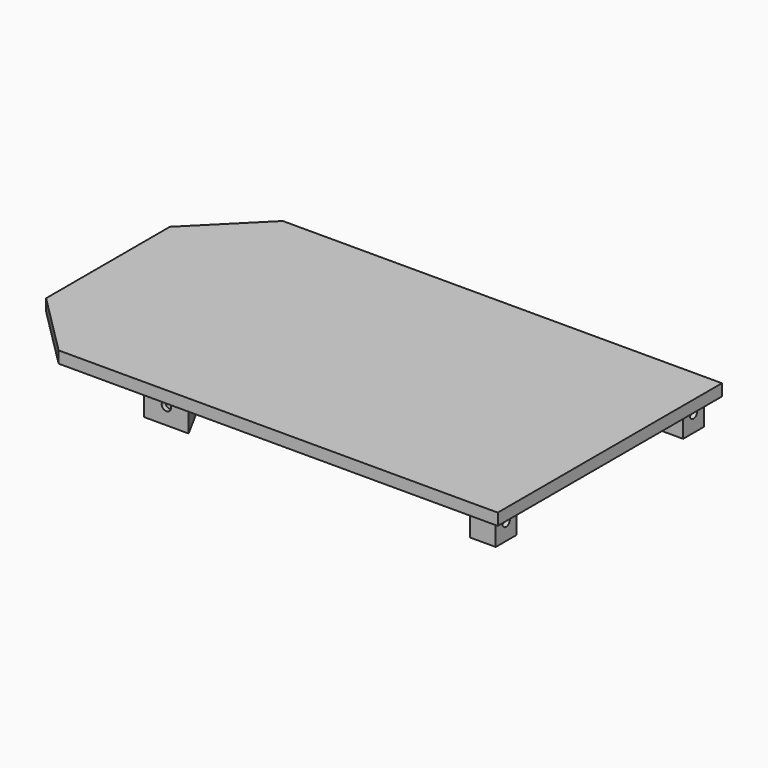
from build123d import *

# Parameters (mm, degrees)
F0_W      = 7.8739928325
F0_H      = 7.8739928325
F1_DEPTH  = 2.54
F2_DEPTH  = 1.016
F3_DEPTH  = 8.89
F8_W      = 2.286
F8_H      = 6.35
F7_W      = 2.286
F7_H      = 6.35
F4_W      = 6.35
F4_H      = 2.286
F5_W      = 2.286
F5_H      = 6.35
F6_W      = 6.35
F6_H      = 2.286
F9_DEPTH  = 8.255
F10_R     = 1.4224
F11_DEPTH = 101.6
F12_R     = 1.4224
F13_R     = 1.4224
F14_DEPTH = 25.4
F15_R     = 1.4224
F16_DEPTH = 25.4


# Not quite as in the source:
# - a feature names something its author has since deleted; it is built from what else it names


with BuildPart() as f1:
    # F0 (on Top) → F1 (new body)
    with BuildSketch(Plane.XY):
        Polygon((-50.5911594971, 45.1345390935), (-65.0638575705, 30.6618410202), (-69.6408525109, 26.0848460797), (-69.6408525109, 9.5127671957), (-69.6408525109, -20.9057678927), (-62.6880467633, -27.8585736403), (-50.5911594971, -39.9554609065), (82.7588405029, -39.9554609065), (82.7588405029, -17.0967224985), (82.7588405029, 43.8645390935), (82.7588405029, 45.1345390935), (33.1444106996, 45.1345390935), (-20.2568043023, 45.1345390935), align=None)
        Polygon((-50.0651082729, -38.6854609065), (-68.3711594971, -20.3794096823), (-68.3711594971, 25.5584878693), (-64.1658319583, 29.763815408), (-50.0651082729, 43.8645390935), (81.4888405029, 43.8645390935), (81.4888405029, -38.6854609065), align=None, mode=Mode.SUBTRACT)
        Polygon((-68.3711594971, 25.5584878693), (-68.3711594971, -20.3794096823), (-50.0651082729, -38.6854609065), (81.4888405029, -38.6854609065), (81.4888405029, 43.8645390935), (-50.0651082729, 43.8645390935), (-64.1658319583, 29.763815408), align=None)
        Polygon((-13.562855112, -36.9074608927), (-27.0518330949, -36.9074608927), (-22.3274411258, -29.0334609202), (-17.8373202542, -29.0334609202), align=None, mode=Mode.SUBTRACT)
        Polygon((-66.5931594971, -19.6429379684), (-66.5931594971, -12.7413552397), (-60.0190392027, -12.7413552397), (-60.413067775, -19.6310556945), (-63.509054773, -22.7270426925), align=None, mode=Mode.SUBTRACT)
        with BuildLine():
            Line((-49.5390570487, -37.4154609065), (-61.7130058245, -25.2415121307))
            Line((-61.7130058245, -25.2415121307), (-58.120903376, -21.6494096823))
            Line((-58.120903376, -21.6494096823), (-56.9411594971, -12.2333584581))
            Line((-56.9411594971, -12.2333584581), (-56.9411594971, -9.6933584581))
            Line((-56.9411594971, -9.6933584581), (-67.1011594971, -9.6933584581))
            Line((-67.1011594971, -9.6933584581), (-67.1011594971, 25.0324366451))
            Line((-67.1011594971, 25.0324366451), (-49.5390570487, 42.5945390935))
            Line((-49.5390570487, 42.5945390935), (-33.3653066841, 42.5945390935))
            ThreePointArc((-33.3653066841, 42.5945390935), (-30.8623950498, 41.9351536832), (-29.0092406655, 40.128174271))
            Line((-29.0092406655, 40.128174271), (-25.1550660971, 33.7045390935))
            ThreePointArc((-25.1550660971, 33.7045390935), (-23.284234992, 31.8649136199), (-20.7556570459, 31.1645390935))
            Line((-20.7556570459, 31.1645390935), (-19.3944751483, 31.1645390935))
            ThreePointArc((-19.3944751483, 31.1645390935), (-16.8544751483, 31.8451300423), (-14.9950660971, 33.7045390935))
            Line((-14.9950660971, 33.7045390935), (-11.6110890868, 39.9381692669))
            ThreePointArc((-11.6110890868, 39.9381692669), (-9.7440488814, 41.8802258253), (-7.1465155593, 42.5945390935))
            Line((-7.1465155593, 42.5945390935), (67.5188405029, 42.5945390935))
            ThreePointArc((67.5188405029, 42.5945390935), (69.3148917271, 41.8505903177), (70.0588405029, 40.0545390935))
            Line((70.0588405029, 40.0545390935), (70.0588405029, 32.4345390935))
            Line((70.0588405029, 32.4345390935), (77.6788405029, 32.4345390935))
            ThreePointArc((77.6788405029, 32.4345390935), (79.4748917271, 31.6905903177), (80.2188405029, 29.8945390935))
            Line((80.2188405029, 29.8945390935), (80.2188405029, -24.7154609065))
            ThreePointArc((80.2188405029, -24.7154609065), (79.4748917271, -26.5115121307), (77.6788405029, -27.2554609065))
            Line((77.6788405029, -27.2554609065), (70.0588405029, -27.2554609065))
            Line((70.0588405029, -27.2554609065), (70.0588405029, -34.8754609065))
            ThreePointArc((70.0588405029, -34.8754609065), (69.3148917271, -36.6715121307), (67.5188405029, -37.4154609065))
            Line((67.5188405029, -37.4154609065), (-7.1465155593, -37.4154609065))
            ThreePointArc((-7.1465155593, -37.4154609065), (-9.7440488814, -36.7011476383), (-11.6110890868, -34.7590910799))
            Line((-11.6110890868, -34.7590910799), (-14.9950660971, -28.5254609065))
            ThreePointArc((-14.9950660971, -28.5254609065), (-16.8544751483, -26.6660518553), (-19.3944751483, -25.9854609065))
            Line((-19.3944751483, -25.9854609065), (-20.7556570459, -25.9854609065))
            ThreePointArc((-20.7556570459, -25.9854609065), (-23.284234992, -26.6858354329), (-25.1550660971, -28.5254609065))
            Line((-25.1550660971, -28.5254609065), (-29.0092406655, -34.949096084))
            ThreePointArc((-29.0092406655, -34.949096084), (-30.8623950498, -36.7560754962), (-33.3653066841, -37.4154609065))
            Line((-33.3653066841, -37.4154609065), (-49.5390570487, -37.4154609065))
        make_face(mode=Mode.SUBTRACT)
        with Locations((75.7738405029, -32.9704609065)):
            Rectangle(F0_W, F0_H, mode=Mode.SUBTRACT)
        Polygon((-27.0518310596, 42.0865379274), (-13.5628570488, 42.0865379274), (-17.8373209399, 34.2125402596), (-22.3274404733, 34.2125402596), align=None, mode=Mode.SUBTRACT)
        with Locations((75.7738405029, 38.1495390935)):
            Rectangle(F0_W, F0_H, mode=Mode.SUBTRACT)
        with BuildLine():
            Line((-58.120903376, -21.6494096823), (-61.7130058245, -25.2415121307))
            Line((-61.7130058245, -25.2415121307), (-49.5390570487, -37.4154609065))
            Line((-49.5390570487, -37.4154609065), (-33.3653066841, -37.4154609065))
            ThreePointArc((-33.3653066841, -37.4154609065), (-30.8623950498, -36.7560754962), (-29.0092406655, -34.949096084))
            Line((-29.0092406655, -34.949096084), (-25.1550660971, -28.5254609065))
            ThreePointArc((-25.1550660971, -28.5254609065), (-23.284234992, -26.6858354329), (-20.7556570459, -25.9854609065))
            Line((-20.7556570459, -25.9854609065), (-19.3944751483, -25.9854609065))
            ThreePointArc((-19.3944751483, -25.9854609065), (-16.8544751483, -26.6660518553), (-14.9950660971, -28.5254609065))
            Line((-14.9950660971, -28.5254609065), (-11.6110890868, -34.7590910799))
            ThreePointArc((-11.6110890868, -34.7590910799), (-9.7440488814, -36.7011476383), (-7.1465155593, -37.4154609065))
            Line((-7.1465155593, -37.4154609065), (67.5188405029, -37.4154609065))
            ThreePointArc((67.5188405029, -37.4154609065), (69.3148917271, -36.6715121307), (70.0588405029, -34.8754609065))
            Line((70.0588405029, -34.8754609065), (70.0588405029, -27.2554609065))
            Line((70.0588405029, -27.2554609065), (77.6788405029, -27.2554609065))
            ThreePointArc((77.6788405029, -27.2554609065), (79.4748917271, -26.5115121307), (80.2188405029, -24.7154609065))
            Line((80.2188405029, -24.7154609065), (80.2188405029, 29.8945390935))
            ThreePointArc((80.2188405029, 29.8945390935), (79.4748917271, 31.6905903177), (77.6788405029, 32.4345390935))
            Line((77.6788405029, 32.4345390935), (70.0588405029, 32.4345390935))
            Line((70.0588405029, 32.4345390935), (70.0588405029, 40.0545390935))
            ThreePointArc((70.0588405029, 40.0545390935), (69.3148917271, 41.8505903177), (67.5188405029, 42.5945390935))
            Line((67.5188405029, 42.5945390935), (-7.1465155593, 42.5945390935))
            ThreePointArc((-7.1465155593, 42.5945390935), (-9.7440488814, 41.8802258253), (-11.6110890868, 39.9381692669))
            Line((-11.6110890868, 39.9381692669), (-14.9950660971, 33.7045390935))
            ThreePointArc((-14.9950660971, 33.7045390935), (-16.8544751483, 31.8451300423), (-19.3944751483, 31.1645390935))
            Line((-19.3944751483, 31.1645390935), (-20.7556570459, 31.1645390935))
            ThreePointArc((-20.7556570459, 31.1645390935), (-23.284234992, 31.8649136199), (-25.1550660971, 33.7045390935))
            Line((-25.1550660971, 33.7045390935), (-29.0092406655, 40.128174271))
            ThreePointArc((-29.0092406655, 40.128174271), (-30.8623950498, 41.9351536832), (-33.3653066841, 42.5945390935))
            Line((-33.3653066841, 42.5945390935), (-49.5390570487, 42.5945390935))
            Line((-49.5390570487, 42.5945390935), (-67.1011594971, 25.0324366451))
            Line((-67.1011594971, 25.0324366451), (-67.1011594971, -9.6933584581))
            Line((-67.1011594971, -9.6933584581), (-56.9411594971, -9.6933584581))
            Line((-56.9411594971, -9.6933584581), (-56.9411594971, -12.2333584581))
            Line((-56.9411594971, -12.2333584581), (-58.120903376, -21.6494096823))
        make_face()
        Polygon((-22.3274411258, -29.0334609202), (-27.0518330949, -36.9074608927), (-13.562855112, -36.9074608927), (-17.8373202542, -29.0334609202), align=None)
        Polygon((-17.8373209399, 34.2125402596), (-13.5628570488, 42.0865379274), (-27.0518310596, 42.0865379274), (-22.3274404733, 34.2125402596), align=None)
        with Locations((75.7738405029, -32.9704609065)):
            Rectangle(F0_W, F0_H)
        with Locations((75.7738405029, 38.1495390935)):
            Rectangle(F0_W, F0_H)
        Polygon((-60.0190392027, -12.7413552397), (-66.5931594971, -12.7413552397), (-66.5931594971, -19.6429379684), (-63.509054773, -22.7270426925), (-60.413067775, -19.6310556945), align=None)
    extrude(amount=F1_DEPTH)

    # F0 (on Top) → F2 (join)
    with BuildSketch(Plane.XY):
        Polygon((-50.5911594971, 45.1345390935), (-65.0638575705, 30.6618410202), (-69.6408525109, 26.0848460797), (-69.6408525109, 9.5127671957), (-69.6408525109, -20.9057678927), (-62.6880467633, -27.8585736403), (-50.5911594971, -39.9554609065), (82.7588405029, -39.9554609065), (82.7588405029, -17.0967224985), (82.7588405029, 43.8645390935), (82.7588405029, 45.1345390935), (33.1444106996, 45.1345390935), (-20.2568043023, 45.1345390935), align=None)
        Polygon((-50.0651082729, -38.6854609065), (-68.3711594971, -20.3794096823), (-68.3711594971, 25.5584878693), (-64.1658319583, 29.763815408), (-50.0651082729, 43.8645390935), (81.4888405029, 43.8645390935), (81.4888405029, -38.6854609065), align=None, mode=Mode.SUBTRACT)
    extrude(amount=-F2_DEPTH)

    # F0 (on Top) → F3 (join)
    with BuildSketch(Plane.XY):
        Polygon((-17.8373209399, 34.2125402596), (-13.5628570488, 42.0865379274), (-27.0518310596, 42.0865379274), (-22.3274404733, 34.2125402596), align=None)
        Polygon((-22.3274411258, -29.0334609202), (-27.0518330949, -36.9074608927), (-13.562855112, -36.9074608927), (-17.8373202542, -29.0334609202), align=None)
        Polygon((-60.0190392027, -12.7413552397), (-66.5931594971, -12.7413552397), (-66.5931594971, -19.6429379684), (-63.509054773, -22.7270426925), (-60.413067775, -19.6310556945), align=None)
        with Locations((75.7738405029, -32.9704609065)):
            Rectangle(F0_W, F0_H)
        with Locations((75.7738405029, 38.1495390935)):
            Rectangle(F0_W, F0_H)
    extrude(amount=-F3_DEPTH)

    # F8 (on face) + F7 (on face) + F4 (on face) + F5 (on face) + F6 (on face) → F9 (cut)
    with BuildSketch(Plane(origin=(0, 0, -8.89), x_dir=(1, 0, 0), z_dir=(0, 0, -1))):
        with Locations((77.1708369192, -38.1495390935)):
            Rectangle(F8_W, F8_H)
    with BuildSketch(Plane(origin=(0, 0, -8.89), x_dir=(1, 0, 0), z_dir=(0, 0, -1))):
        with Locations((77.1708369192, 32.9704609065)):
            Rectangle(F7_W, F7_H)
    with BuildSketch(Plane(origin=(0, 0, -8.89), x_dir=(1, 0, 0), z_dir=(0, 0, -1))):
        with Locations((-20.3073441034, 34.3674608927)):
            Rectangle(F4_W, F4_H)
    with BuildSketch(Plane(origin=(0, 0, -8.89), x_dir=(1, 0, 0), z_dir=(0, 0, -1))):
        with Locations((-64.0531594971, 16.9871170074)):
            Rectangle(F5_W, F5_H)
    with BuildSketch(Plane(origin=(0, 0, -8.89), x_dir=(1, 0, 0), z_dir=(0, 0, -1))):
        with Locations((-20.3073440542, -39.5465379274)):
            Rectangle(F6_W, F6_H)
    extrude(amount=-F9_DEPTH, mode=Mode.SUBTRACT)

    # F10 (on face) → F11 (cut)
    with BuildSketch(Plane(origin=(0, 42.0865379274, 0), x_dir=(-1, 0, 0), z_dir=(0, 1, 0))):
        with Locations((20.3073440542, -3.683)):
            Circle(F10_R)
    extrude(amount=-F11_DEPTH, mode=Mode.SUBTRACT)

    # F12 (on face) + F13 (on face) → F14 (cut)
    with BuildSketch(Plane.YZ.offset(79.7108369192)):
        with Locations((38.1495390935, -3.683)):
            Circle(F12_R)
    with BuildSketch(Plane.YZ.offset(79.7108369192)):
        with Locations((-32.9704609065, -3.683)):
            Circle(F13_R)
    extrude(amount=-F14_DEPTH, mode=Mode.SUBTRACT)

    # F15 (on face) → F16 (cut)
    with BuildSketch(Plane(origin=(-66.5931594971, 0, 0), x_dir=(0, -1, 0), z_dir=(-1, 0, 0))):
        with Locations((16.9831552397, -3.683)):
            Circle(F15_R)
    extrude(amount=-F16_DEPTH, mode=Mode.SUBTRACT)


solid = f1.part
